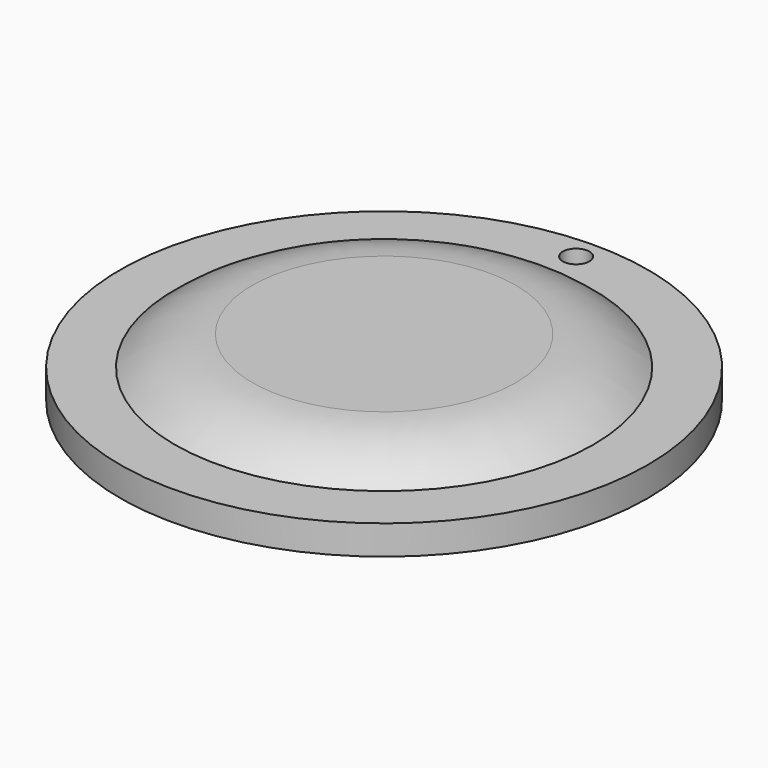
from build123d import *

# Parameters (mm, degrees)
F0_R     = 28.575
F2_DEPTH = 3.175
F1_R     = 22.6695
F3_DEPTH = 6.35
F4_R     = 1.4432349382
F5_DEPTH = 6.351


# Not quite as in the source:
# - a fillet or chamfer that OpenCascade refuses, or shapes differently, is made with other operations: its cross-section is extruded or revolved along the edge and cut away or added


with BuildPart() as f2:
    # F0 (on Top) → F2 (new body)
    with BuildSketch(Plane.XY):
        Circle(F0_R)
    extrude(amount=F2_DEPTH)

    # F1 (on Top) → F3 (join)
    with BuildSketch(Plane.XY):
        Circle(F1_R)
    extrude(amount=F3_DEPTH)

    # F4 (on face) → F5 (cut, through all)
    with BuildSketch(Plane.XY.offset(6.35)):
        with Locations((0, 25.9878132492)):
            Circle(F4_R)
    extrude(amount=-F5_DEPTH, mode=Mode.SUBTRACT)

    # F6: fillet of radius 12.7 on 1 edges, made by hand

    # F6_s1 → F6_t2 (revolve, cut)
    with BuildSketch(Plane.XZ):
        with BuildLine():
            ThreePointArc((22.6695, 3.175), (18.7593676479, 5.529762203), (14.2692395874, 6.35))
            Line((14.2692395874, 6.35), (14.2692395874, 6.604))
            Line((14.2692395874, 6.604), (22.6695, 6.604))
            Line((22.6695, 6.604), (22.9235, 6.35))
            ThreePointArc((22.9235, 6.35), (22.9235, 4.7625), (22.8375052083, 3.3655))
            Line((22.8375052083, 3.3655), (22.6695, 3.175))
        make_face()
    revolve(axis=Axis((0, 0, 6.35), (0, 0, 1)), mode=Mode.SUBTRACT)


solid = f2.part
